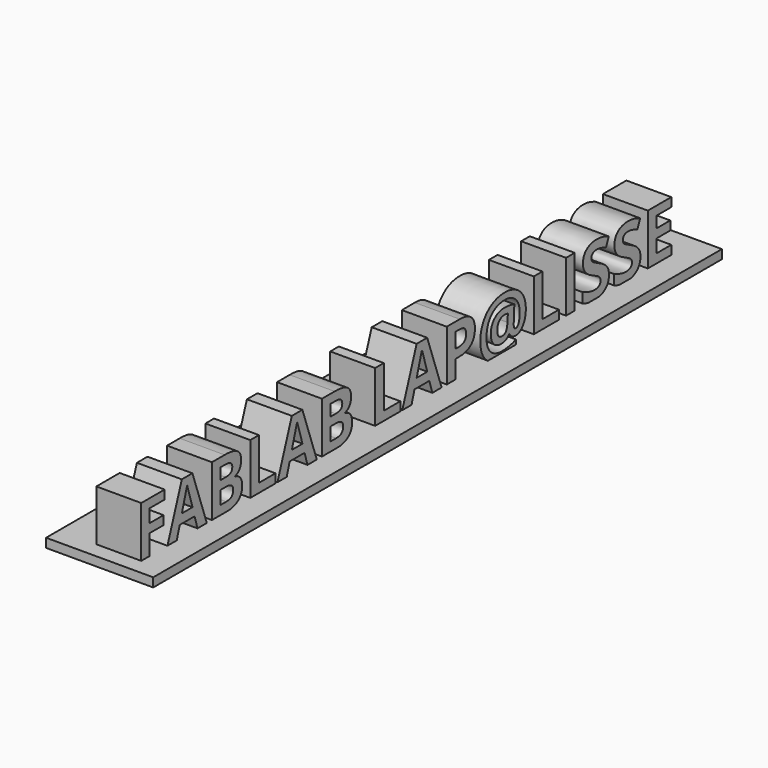
from build123d import *

# Parameters (mm, degrees)
F0_TEXT_SIZE = 15.8882526232
F1_DEPTH     = 10
F2_W         = 23.8596154377
F2_H         = 158.2996007055
F3_DEPTH     = 2


# Not quite as in the source:
# - Text() gives the source's letters only with a copy of the font that has no kerning and outlines rounded to 1/6400 em; it was checked with that copy


with BuildPart() as f1:
    # F0 (on Right) → F1 (new body)
    with BuildSketch(Plane.YZ):
        with Locations((-12.1958065735, 0)):
            Text('FABLAB LAP@LISSE', F0_TEXT_SIZE, font='Open Sans', font_style=FontStyle.BOLD, text_align=(TextAlign.LEFT, TextAlign.BOTTOM))
    extrude(amount=F1_DEPTH)


with BuildPart() as f3:
    # F2 (on Top) → F3 (new body)
    with BuildSketch(Plane.XY):
        with Locations((3.5605705343, 64.853859134)):
            Rectangle(F2_W, F2_H)
    extrude(amount=-F3_DEPTH)


solid = Compound([f1.part, f3.part])
